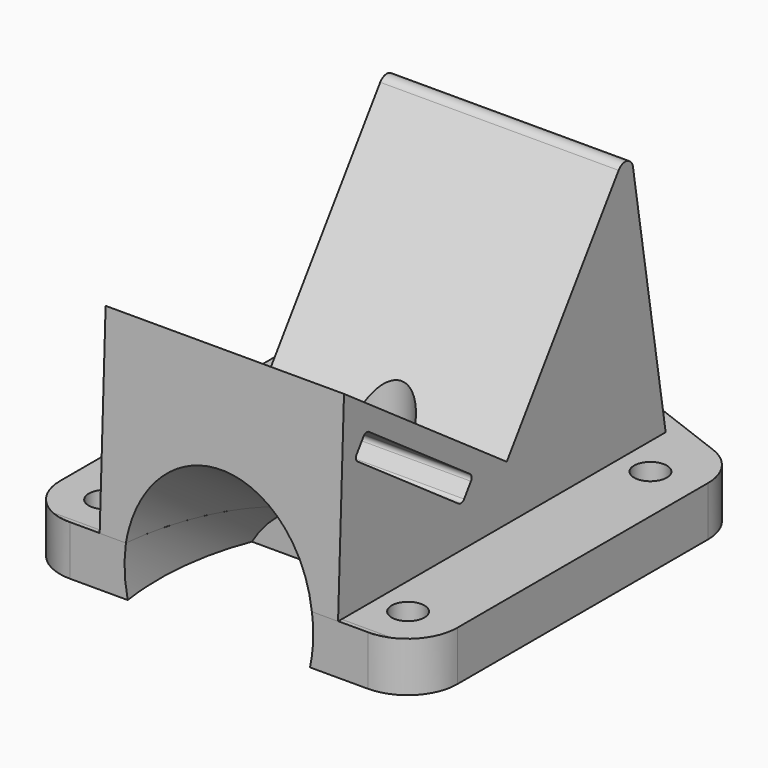
from build123d import *

# Parameters (mm, degrees)
F0_R          = 1.65
F0_R_2        = 3.5
F1_DEPTH      = 5
F3_DEPTH      = 40
F4_R          = 9.5
F5_DEPTH      = 25
F6_R          = 1.675
F7_DEPTH      = 25
F7_DEPTH_BACK = 25
F8_R          = 3
F9_DEPTH      = 40
F11_DEPTH     = 40
F12_W         = 9.1582505405
F12_H         = 40
F12_W_2       = 8.5622543842
F13_DEPTH     = 50
F14_R         = 1
F15_R         = 4.875
F16_DEPTH     = 2.5
F17_W         = 15.5204893433
F17_H         = 2.5680447786
F18_DEPTH     = 5


with BuildPart() as f1:
    # F0 (on Top) → F1 (new body)
    with BuildSketch(Plane.XY):
        with BuildLine():
            Line((-15, -20), (15, -20))
            ThreePointArc((15, -20), (18.5355339059, -18.5355339059), (20, -15))
            Line((20, -15), (20, 16.5542368918))
            ThreePointArc((20, 16.5542368918), (19.643027324, 18.4095797898), (18.6230810925, 20))
            Line((18.6230810925, 20), (-19.6336355125, 20))
            ThreePointArc((-19.6336355125, 20), (-19.9075542566, 19.078356926), (-20, 18.1213244195))
            Line((-20, 18.1213244195), (-20, -15))
            ThreePointArc((-20, -15), (-18.5355339059, -18.5355339059), (-15, -20))
        make_face()
        with Locations((-15.25, -15.25)):
            Circle(F0_R, mode=Mode.SUBTRACT)
        with Locations((15.25, -15.25)):
            Circle(F0_R, mode=Mode.SUBTRACT)
        with Locations((-15.25, 15.25)):
            Circle(F0_R, mode=Mode.SUBTRACT)
        with Locations((15.25, 15.25)):
            Circle(F0_R, mode=Mode.SUBTRACT)
        with BuildLine():
            Line((-19.6336355125, 20), (18.6230810925, 20))
            ThreePointArc((18.6230810925, 20), (17.7702782254, 20.7166350653), (16.779976638, 21.2266755665))
            Line((16.779976638, 21.2266755665), (-1, 28))
            ThreePointArc((-1, 28), (-7, 22), (-13, 28))
            Line((-13, 28), (-18.7628834735, 21.4138474588))
            ThreePointArc((-18.7628834735, 21.4138474588), (-19.2573611463, 20.7433229072), (-19.6336355125, 20))
        make_face()
        with BuildLine():
            ThreePointArc((-13, 28), (-7, 22), (-1, 28))
            ThreePointArc((-1, 28), (-7, 34), (-13, 28))
        make_face()
        with Locations((-7, 28)):
            Circle(F0_R_2, mode=Mode.SUBTRACT)
    extrude(amount=F1_DEPTH)


with BuildPart() as f3:
    # F2 (on face) → F3 (new body)
    with BuildSketch(Plane.YZ.offset(20)):
        Polygon((1.2266755665, 10.51673083), (-19.2521255407, 24.8561417388), (-20, 5), (21.2266755665, 5), (16.713239348, 32.6338360258), align=None)
        with BuildLine():
            ThreePointArc((-16.7950944212, 20.0837735554), (-16.4723424879, 20.2893892137), (-16.0987301809, 20.2065613594))
            Line((-16.0987301809, 20.2065613594), (-3.4018734944, 11.3161265959))
            ThreePointArc((-3.4018734944, 11.3161265959), (-3.1962578361, 10.9933746626), (-3.2790856905, 10.6197623556))
            Line((-3.2790856905, 10.6197623556), (-4.139450345, 9.3910342892))
            ThreePointArc((-4.139450345, 9.3910342892), (-4.4622022783, 9.1854186308), (-4.8358145853, 9.2682464852))
            Line((-4.8358145853, 9.2682464852), (-17.5326712718, 18.1586812486))
            ThreePointArc((-17.5326712718, 18.1586812486), (-17.7382869301, 18.481433182), (-17.6554590758, 18.855045489))
            Line((-17.6554590758, 18.855045489), (-16.7950944212, 20.0837735554))
        make_face(mode=Mode.SUBTRACT)
    extrude(amount=-F3_DEPTH)


with BuildPart() as f5_tool:
    # F4 (on face) → F5 (new body)
    with BuildSketch(Plane(origin=(0, -4.1181355181, 2.8835495331), x_dir=(1, 0, 0), z_dir=(0, -0.8191520443, 0.5735764364))):
        with Locations((0, -9)):
            Circle(F4_R)
    extrude(amount=F5_DEPTH)


with BuildPart() as f1_1:
    add(f1.part)

    # F5: cut by f5_tool
    add(f5_tool.part, mode=Mode.SUBTRACT)


with BuildPart() as f3_1:
    add(f3.part)

    # F5: cut by f5_tool
    add(f5_tool.part, mode=Mode.SUBTRACT)


with BuildPart() as f7_tool:
    # F6 (on face) → F7 (new body, two sides)
    with BuildSketch(Plane.XY.offset(5)) as f7_sk:
        Circle(F6_R)
    extrude(amount=F7_DEPTH)
    extrude(f7_sk.sketch, amount=-F7_DEPTH_BACK)


with BuildPart() as f1_2:
    add(f1_1.part)

    # F7: cut by f7_tool
    add(f7_tool.part, mode=Mode.SUBTRACT)

    # F15 (on face) → F16 (cut)
    with BuildSketch(Plane.XY.offset(5)):
        with Locations((-7, 28)):
            Circle(F15_R)
    extrude(amount=-F16_DEPTH, mode=Mode.SUBTRACT)


with BuildPart() as f3_2:
    add(f3_1.part)

    # F7: cut by f7_tool
    add(f7_tool.part, mode=Mode.SUBTRACT)

    # F8 (on face) → F9 (cut)
    with BuildSketch(Plane.XY.offset(5)):
        with Locations((-15.25, -15.25)):
            Circle(F8_R)
        with Locations((-15.25, 15.25)):
            Circle(F8_R)
        with Locations((15.25, 15.25)):
            Circle(F8_R)
        with Locations((15.25, -15.25)):
            Circle(F8_R)
        Circle(F8_R)
    extrude(amount=F9_DEPTH, mode=Mode.SUBTRACT)

    # F10 (on face) → F11 (cut)
    with BuildSketch(Plane(origin=(0, 0, 0), x_dir=(1, 0, 0), z_dir=(0, 0, -1))):
        with BuildLine():
            ThreePointArc((-20, 15), (-18.5355339059, 18.5355339059), (-15, 20))
            Line((-15, 20), (-18.4092409909, 22.2686175257))
            Line((-18.4092409909, 22.2686175257), (-22.4427245557, 20.613854751))
            Line((-22.4427245557, 20.613854751), (-20, 15))
        make_face()
        with BuildLine():
            Line((15.3065547347, 23.8199587911), (15, 20))
            ThreePointArc((15, 20), (18.5355339059, 18.5355339059), (20, 15))
            Line((20, 15), (20, 23.8199587911))
            Line((20, 23.8199587911), (15.3065547347, 23.8199587911))
        make_face()
    extrude(amount=-F11_DEPTH, mode=Mode.SUBTRACT)

    # F12 (on face) → F13 (cut)
    with BuildSketch(Plane(origin=(0, -20.1597241143, 0.7593087806), x_dir=(1, 0, 0), z_dir=(0, -0.9992914412, 0.0376379538))):
        with Locations((16.5791252702, 24.2608358153)):
            Rectangle(F12_W, F12_H)
        with Locations((-16.2811271921, 24.2608358153)):
            Rectangle(F12_W_2, F12_H)
    extrude(amount=-F13_DEPTH, mode=Mode.SUBTRACT)

    # F14
    f14_edges = [f3_2.edges().sort_by_distance(p)[0] for p in [
        (0, 16.713239, 32.633836),
    ]]
    fillet(f14_edges, radius=F14_R)


with BuildPart() as f18:
    # F17 (on face) → F18 (new body)
    with BuildSketch(Plane(origin=(0, 0, 0), x_dir=(1, 0, 0), z_dir=(0, 0, -1))):
        with Locations((0, 4.8531962487)):
            Rectangle(F17_W, F17_H)
    extrude(amount=-F18_DEPTH)


solid = Compound([f1_2.part, f3_2.part, f18.part])
